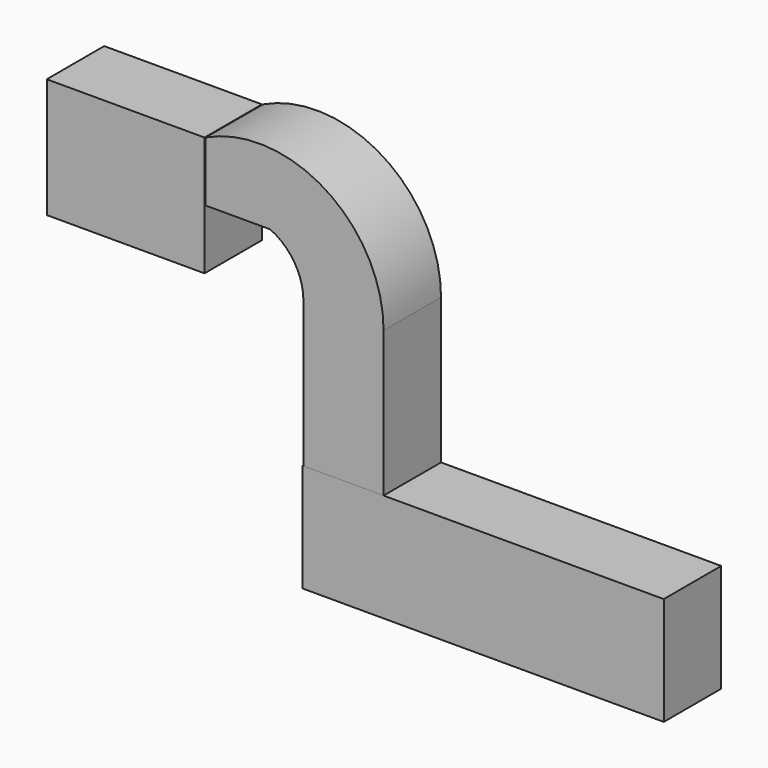
from build123d import *

# Parameters (mm, degrees)
F0_W     = 127.7624070644
F0_H     = 38.2387563586
F2_DEPTH = 25.4
F0_W_2   = 55.7835698128
F0_H_2   = 42.2875583172
F3_DEPTH = 25.4


with BuildPart() as f2:
    # F0 (on Front) → F2 (new body)
    with BuildSketch(Plane.XZ):
        Rectangle(F0_W, F0_H)
    extrude(amount=F2_DEPTH)


with BuildPart() as f2b:
    # F0 (on Front) → F2, piece 2 (new body)
    with BuildSketch(Plane.XZ):
        with Locations((-126.4128237963, 88.8488590717)):
            Rectangle(F0_W_2, F0_H_2)
    extrude(amount=F2_DEPTH)


with BuildPart() as f2c:
    # F1 (on Front) → F2, piece 3 (new body)
    with BuildSketch(Plane.XZ):
        with BuildLine():
            Line((-63.5438114405, 70.5167576671), (-63.5438114405, 19.0069098026))
            Line((-63.5438114405, 19.0069098026), (-35.2021455765, 19.0069098026))
            Line((-35.2021455765, 19.0069098026), (-35.2021455765, 70.5167576671))
            ThreePointArc((-35.2021455765, 70.5167576671), (-55.755160611, 107.7118696892), (-98.183631897, 110.105112195))
            Line((-98.183631897, 110.105112195), (-98.183631897, 88.9613330364))
            Line((-98.183631897, 88.9613330364), (-75.2403661609, 88.9613330364))
            ThreePointArc((-75.2403661609, 88.9613330364), (-66.7144537907, 81.437057032), (-63.5438114405, 70.5167576671))
        make_face()
    extrude(amount=F2_DEPTH)


with BuildPart() as f3:
    # F0 (on Front) → F3 (new body)
    with BuildSketch(Plane.XZ):
        Rectangle(F0_W, F0_H)
    extrude(amount=F3_DEPTH)


with BuildPart() as f3b:
    # F0 (on Front) → F3, piece 2 (new body)
    with BuildSketch(Plane.XZ):
        with Locations((-126.4128237963, 88.8488590717)):
            Rectangle(F0_W_2, F0_H_2)
    extrude(amount=F3_DEPTH)


solid = Compound([f2.part, f2b.part, f2c.part, f3.part, f3b.part])
